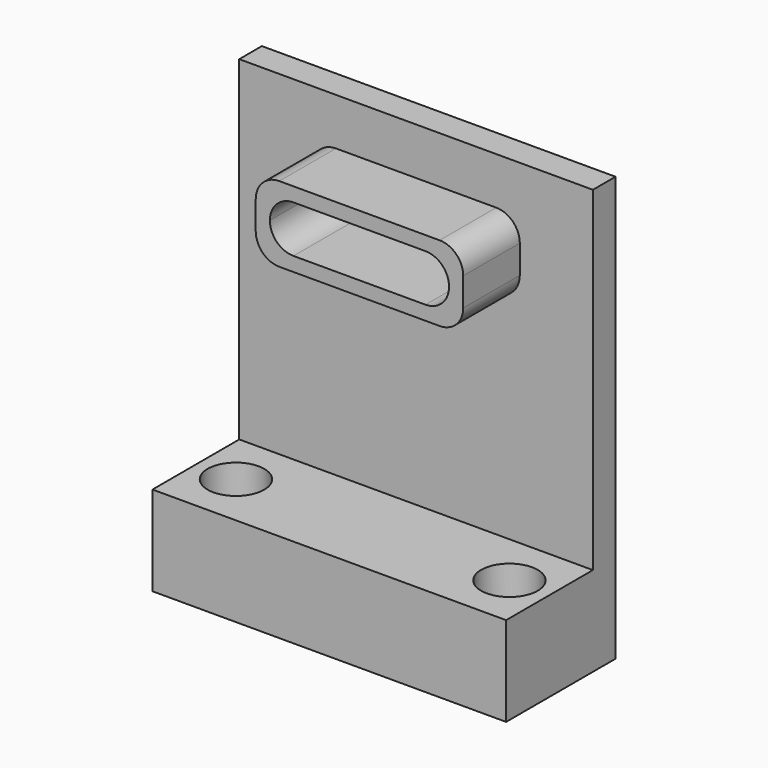
from build123d import *

# Parameters (mm, degrees)
F1_W        = 75
F1_H        = 90
F2_DEPTH    = 6
F3_W        = 75
F3_H        = 19
F4_DEPTH    = 23
F5_R        = 6
F6_DEPTH    = 19
F7_W        = 44
F7_H        = 16
F8_DEPTH    = 15
F9_T        = 3
F9_T3_DEPTH = 81
F9_T5_DEPTH = 22
F9_T7_DEPTH = 50
F10_R       = 4.99999
F11_W       = 20
F11_H       = 10
F12_DEPTH   = 20
F13_R       = 7.5
F14_DEPTH   = 40
F15_R       = 5


# Not quite as in the source:
# - a fillet or chamfer is up to 0.001 mm smaller than in the source, because OpenCascade refuses the exact size
# - a shell that OpenCascade refuses in one call is made with other operations: the cavity is built on its own and cut out


with BuildPart() as f2:
    # F1 (on Front) → F2 (new body)
    with BuildSketch(Plane.XZ):
        with Locations((2.5936549902, -11.7762294412)):
            Rectangle(F1_W, F1_H)
    extrude(amount=F2_DEPTH)

    # F3 (on face) → F4 (join)
    with BuildSketch(Plane.XZ.offset(6)):
        with Locations((2.5936549902, -47.2762294412)):
            Rectangle(F3_W, F3_H)
    extrude(amount=F4_DEPTH)

    # F5 (on face) → F6 (cut, through all)
    with BuildSketch(Plane.XY.offset(-37.7762294412)):
        with Locations((-26.4063450098, -17.5)):
            Circle(F5_R)
        with Locations((31.5936549902, -17.5)):
            Circle(F5_R)
    extrude(amount=-F6_DEPTH, mode=Mode.SUBTRACT)

    # F7 (on face) → F8 (join)
    with BuildSketch(Plane.XZ.offset(6)):
        with Locations((2.5936549902, 15.2237705588)):
            Rectangle(F7_W, F7_H)
    extrude(amount=F8_DEPTH)

    # F9: shell of thickness 3, made by hand


with BuildPart() as f9_core1:
    # F9_t2: copy of F2
    add(f2.part)

    # the walls: a layer under each face that stays
    f9_faces = [f9_core1.faces().sort_by_distance(p)[0] for p in [
        (40.0936549902, -24.1666666667, -41.7762294412),
        (2.5936549902, -14.5, -56.7762294412),
        (2.5936549902, -29, -47.2762294412),
        (2.5936549902, -17.5, -37.7762294412),
        (2.5936549902, -6, -2.2762294412),
        (2.5936549902, -3, 33.2237705588),
        (2.5936549902, 0, -11.7762294412),
        (-34.9063450098, -4.8333333333, 18.2237705588),
        (-32.4063450098, -17.5, -47.2762294412),
        (25.5936549902, -17.5, -47.2762294412),
        (24.5936549902, -13.5, 15.2237705588),
        (2.5936549902, -13.5, 23.2237705588),
        (-19.4063450098, -13.5, 15.2237705588),
        (2.5936549902, -13.5, 7.2237705588),
    ]]
    thicken(f9_faces, amount=-F9_T, mode=Mode.SUBTRACT)

    # F9_s4 → F9_t3 (cut)
    with BuildSketch(Plane.YZ.offset(-37.9063450098)):
        Polygon((-6.03, -37.7462294412), (-6, -40.7762294412), (-3, -40.7762294412), (-3, -37.7762294412), align=None)
    extrude(amount=F9_T3_DEPTH, mode=Mode.SUBTRACT)

    # F9_s6 → F9_t5 (cut)
    with BuildSketch(Plane.XY.offset(4.2237705588)):
        Polygon((24.6236549902, -6.03), (24.5936549902, -3), (21.5936549902, -3), (21.5936549902, -6), align=None)
        Polygon((-19.4363450098, -6.03), (-19.4063450098, -3), (-16.4063450098, -3), (-16.4063450098, -6), align=None)
    extrude(amount=F9_T5_DEPTH, mode=Mode.SUBTRACT)

    # F9_s8 → F9_t7 (cut)
    with BuildSketch(Plane.YZ.offset(-22.4063450098)):
        Polygon((-6.03, 23.2537705588), (-3, 23.2237705588), (-3, 20.2237705588), (-6, 20.2237705588), align=None)
        Polygon((-6.03, 7.1937705588), (-3, 7.2237705588), (-3, 10.2237705588), (-6, 10.2237705588), align=None)
    extrude(amount=F9_T7_DEPTH, mode=Mode.SUBTRACT)


with BuildPart() as f2_1:
    add(f2.part)

    # what is left inside the walls is the cavity
    f9_cavity = [f9_core1.part.solids().sort_by_distance(p)[0] for p in [
        (35.892563, -25.441051, -49.442896),
        (-30.705253, -25.441051, -49.442896),
        (2.593655, -18.333333, -40.806229),
        (2.593655, -15, 10.253771),
    ]]
    add(f9_cavity, mode=Mode.SUBTRACT)

    # F10 (radius 5 in the source; OpenCascade refuses exactly that, so slightly less here)
    f10_edges = [f2_1.edges().sort_by_distance(p)[0] for p in [
        (-19.406345, -13.5, 23.223771),
        (-16.406345, -13.5, 20.223771),
        (-16.406345, -13.5, 10.223771),
        (-19.406345, -13.5, 7.223771),
        (21.593655, -13.5, 20.223771),
        (21.593655, -13.5, 10.223771),
        (24.593655, -13.5, 7.223771),
        (24.593655, -13.5, 23.223771),
    ]]
    fillet(f10_edges, radius=F10_R)

    # F11 (on face) → F12 (join)
    with BuildSketch(Plane(origin=(0, 0, 0), x_dir=(-1, 0, 0), z_dir=(0, 1, 0))):
        with Locations((-2.5936549902, -11.7762294412)):
            Rectangle(F11_W, F11_H)
        with Locations((-2.5936549902, -41.7762294412)):
            Rectangle(F11_W, F11_H)
    extrude(amount=F12_DEPTH)

    # F13 (on face) → F14 (cut, through all)
    with BuildSketch(Plane.XY.offset(-6.7762294412)):
        with Locations((2.5936549902, 10)):
            Circle(F13_R)
    extrude(amount=-F14_DEPTH, mode=Mode.SUBTRACT)

    # F15
    f15_edges = [f2_1.edges().sort_by_distance(p)[0] for p in [
        (12.593655, 20, -11.776229),
        (-7.406345, 20, -11.776229),
        (-7.406345, 0, -11.776229),
        (12.593655, 0, -11.776229),
        (12.593655, 0, -41.776229),
        (12.593655, 20, -41.776229),
        (-7.406345, 0, -41.776229),
        (-7.406345, 20, -41.776229),
    ]]
    fillet(f15_edges, radius=F15_R)


solid = f2_1.part
